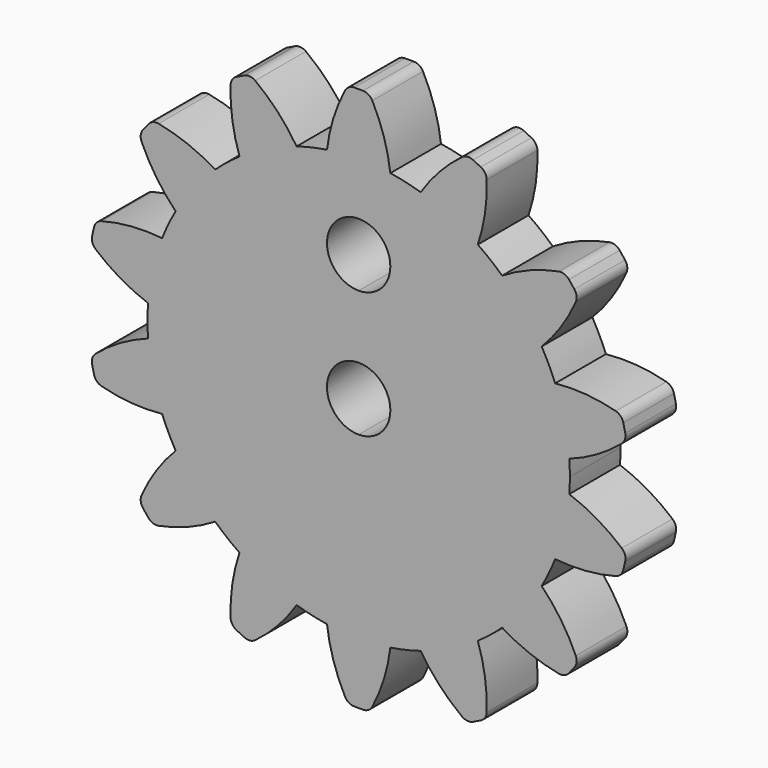
from build123d import *

# Parameters (mm, degrees)
F1_DEPTH = 3
F2_R     = 0.5


# Not quite as in the source:
# - a feature names something its author has since deleted; it is built from what else it names


with BuildPart() as f1:
    # F0 (on Front) → F1 (new body)
    with BuildSketch(Plane.XZ):
        with BuildLine():
            ThreePointArc((9.9727571462, -0.7376414454), (9.9931869657, -0.3690721728), (10, 0))
            ThreePointArc((10, 0), (9.9931869657, 0.3690721728), (9.9727571462, 0.7376414454))
            ThreePointArc((9.9727571462, 0.7376414454), (9.7492791218, 2.2252093396), (9.3051943444, 3.6624251819))
            ThreePointArc((9.3051943444, 3.6624251819), (9.009688679, 4.3388373912), (8.6650930875, 4.9916091379))
            ThreePointArc((8.6650930875, 4.9916091379), (7.8183148247, 6.2348980186), (6.7946236819, 7.3371035853))
            ThreePointArc((6.7946236819, 7.3371035853), (6.2348980186, 7.8183148247), (5.6412010723, 8.2569274226))
            ThreePointArc((5.6412010723, 8.2569274226), (4.3388373912, 9.009688679), (2.9382944686, 9.5585786399))
            ThreePointArc((2.9382944686, 9.5585786399), (2.2252093396, 9.7492791218), (1.5, 9.8868599666))
            ThreePointArc((1.5, 9.8868599666), (0, 10), (-1.5, 9.8868599666))
            ThreePointArc((-1.5, 9.8868599666), (-2.2252093396, 9.7492791218), (-2.9382944686, 9.5585786399))
            ThreePointArc((-2.9382944686, 9.5585786399), (-4.3388373912, 9.009688679), (-5.6412010723, 8.2569274226))
            ThreePointArc((-5.6412010723, 8.2569274226), (-6.2348980186, 7.8183148247), (-6.7946236819, 7.3371035853))
            ThreePointArc((-6.7946236819, 7.3371035853), (-7.8183148247, 6.2348980186), (-8.6650930875, 4.9916091379))
            ThreePointArc((-8.6650930875, 4.9916091379), (-9.009688679, 4.3388373912), (-9.3051943444, 3.6624251819))
            ThreePointArc((-9.3051943444, 3.6624251819), (-9.7492791218, 2.2252093396), (-9.9727571462, 0.7376414454))
            ThreePointArc((-9.9727571462, 0.7376414454), (-10, 0), (-9.9727571462, -0.7376414454))
            ThreePointArc((-9.9727571462, -0.7376414454), (-9.7492791218, -2.2252093396), (-9.3051943444, -3.6624251819))
            ThreePointArc((-9.3051943444, -3.6624251819), (-9.009688679, -4.3388373912), (-8.6650930875, -4.9916091379))
            ThreePointArc((-8.6650930875, -4.9916091379), (-7.8183148247, -6.2348980186), (-6.7946236819, -7.3371035853))
            ThreePointArc((-6.7946236819, -7.3371035853), (-6.2348980186, -7.8183148247), (-5.6412010723, -8.2569274226))
            ThreePointArc((-5.6412010723, -8.2569274226), (-4.3388373912, -9.009688679), (-2.9382944686, -9.5585786399))
            ThreePointArc((-2.9382944686, -9.5585786399), (-2.2252093396, -9.7492791218), (-1.5, -9.8868599666))
            ThreePointArc((-1.5, -9.8868599666), (0, -10), (1.5, -9.8868599666))
            ThreePointArc((1.5, -9.8868599666), (2.2252093396, -9.7492791218), (2.9382944686, -9.5585786399))
            ThreePointArc((2.9382944686, -9.5585786399), (4.3388373912, -9.009688679), (5.6412010723, -8.2569274226))
            ThreePointArc((5.6412010723, -8.2569274226), (6.2348980186, -7.8183148247), (6.7946236819, -7.3371035853))
            ThreePointArc((6.7946236819, -7.3371035853), (7.8183148247, -6.2348980186), (8.6650930875, -4.9916091379))
            ThreePointArc((8.6650930875, -4.9916091379), (9.009688679, -4.3388373912), (9.3051943444, -3.6624251819))
            ThreePointArc((9.3051943444, -3.6624251819), (9.7492791218, -2.2252093396), (9.9727571462, -0.7376414454))
        make_face()
        with BuildLine():
            ThreePointArc((0, 1.5), (1.0606601718, 1.0606601718), (1.5, 0))
            ThreePointArc((1.5, 0), (1.0606601718, -1.0606601718), (0, -1.5))
            ThreePointArc((0, -1.5), (-1.5, 0), (0, 1.5))
        make_face(mode=Mode.SUBTRACT)
        with BuildLine():
            ThreePointArc((1.5, 6), (1.0606601718, 4.9393398282), (0, 4.5))
            ThreePointArc((0, 4.5), (-1.0606601718, 7.0606601718), (1.5, 6))
        make_face(mode=Mode.SUBTRACT)
        with BuildLine():
            ThreePointArc((-5.6412010723, 8.2569274226), (-4.3388373912, 9.009688679), (-2.9382944686, 9.5585786399))
            ThreePointArc((-2.9382944686, 9.5585786399), (-3.9281759427, 10.8096541208), (-5.1466158007, 11.8394402655))
            Line((-5.1466158007, 11.8394402655), (-6.0475846686, 11.4055565264))
            ThreePointArc((-6.0475846686, 11.4055565264), (-6.002150266, 9.8108807266), (-5.6412010723, 8.2569274226))
        make_face()
        with BuildLine():
            ThreePointArc((-1.5, 9.8868599666), (0, 10), (1.5, 9.8868599666))
            ThreePointArc((1.5, 9.8868599666), (1.1509689165, 11.4435335015), (0.5, 12.9))
            Line((0.5, 12.9), (-0.5, 12.9))
            ThreePointArc((-0.5, 12.9), (-1.1509689165, 11.4435335015), (-1.5, 9.8868599666))
        make_face()
        with BuildLine():
            ThreePointArc((-8.6650930875, 4.9916091379), (-7.8183148247, 6.2348980186), (-6.7946236819, 7.3371035853))
            ThreePointArc((-6.7946236819, 7.3371035853), (-8.2292973805, 8.0347901697), (-9.7738812229, 8.4339341852))
            Line((-9.7738812229, 8.4339341852), (-10.3973710248, 7.6521027027))
            ThreePointArc((-10.3973710248, 7.6521027027), (-9.6645321438, 6.2350627012), (-8.6650930875, 4.9916091379))
        make_face()
        with BuildLine():
            ThreePointArc((-9.9727571462, 0.7376414454), (-9.7492791218, 2.2252093396), (-9.3051943444, 3.6624251819))
            ThreePointArc((-9.3051943444, 3.6624251819), (-10.9005055464, 3.6685374852), (-12.4653096002, 3.3579840041))
            Line((-12.4653096002, 3.3579840041), (-12.6878305341, 2.3830560919))
            ThreePointArc((-12.6878305341, 2.3830560919), (-11.4127349029, 1.4243140398), (-9.9727571462, 0.7376414454))
        make_face()
        with BuildLine():
            ThreePointArc((-12.4653096002, -3.3579840041), (-10.9005055464, -3.6685374852), (-9.3051943444, -3.6624251819))
            ThreePointArc((-9.3051943444, -3.6624251819), (-9.7492791218, -2.2252093396), (-9.9727571462, -0.7376414454))
            ThreePointArc((-9.9727571462, -0.7376414454), (-11.4127349029, -1.4243140398), (-12.6878305341, -2.3830560919))
            Line((-12.6878305341, -2.3830560919), (-12.4653096002, -3.3579840041))
        make_face()
        with BuildLine():
            ThreePointArc((-9.7738812229, -8.4339341852), (-8.2292973805, -8.0347901697), (-6.7946236819, -7.3371035853))
            ThreePointArc((-6.7946236819, -7.3371035853), (-7.8183148247, -6.2348980186), (-8.6650930875, -4.9916091379))
            ThreePointArc((-8.6650930875, -4.9916091379), (-9.6645321438, -6.2350627012), (-10.3973710248, -7.6521027027))
            Line((-10.3973710248, -7.6521027027), (-9.7738812229, -8.4339341852))
        make_face()
        with BuildLine():
            ThreePointArc((-5.1466158007, -11.8394402655), (-3.9281759427, -10.8096541208), (-2.9382944686, -9.5585786399))
            ThreePointArc((-2.9382944686, -9.5585786399), (-4.3388373912, -9.009688679), (-5.6412010723, -8.2569274226))
            ThreePointArc((-5.6412010723, -8.2569274226), (-6.002150266, -9.8108807266), (-6.0475846686, -11.4055565264))
            Line((-6.0475846686, -11.4055565264), (-5.1466158007, -11.8394402655))
        make_face()
        with BuildLine():
            ThreePointArc((0.5, -12.9), (1.1509689165, -11.4435335015), (1.5, -9.8868599666))
            ThreePointArc((1.5, -9.8868599666), (0, -10), (-1.5, -9.8868599666))
            ThreePointArc((-1.5, -9.8868599666), (-1.1509689165, -11.4435335015), (-0.5, -12.9))
            Line((-0.5, -12.9), (0.5, -12.9))
        make_face()
        with BuildLine():
            ThreePointArc((6.0475846686, -11.4055565264), (6.002150266, -9.8108807266), (5.6412010723, -8.2569274226))
            ThreePointArc((5.6412010723, -8.2569274226), (4.3388373912, -9.009688679), (2.9382944686, -9.5585786399))
            ThreePointArc((2.9382944686, -9.5585786399), (3.9281759427, -10.8096541208), (5.1466158007, -11.8394402655))
            Line((5.1466158007, -11.8394402655), (6.0475846686, -11.4055565264))
        make_face()
        with BuildLine():
            ThreePointArc((10.3973710248, -7.6521027027), (9.6645321438, -6.2350627012), (8.6650930875, -4.9916091379))
            ThreePointArc((8.6650930875, -4.9916091379), (7.8183148247, -6.2348980186), (6.7946236819, -7.3371035853))
            ThreePointArc((6.7946236819, -7.3371035853), (8.2292973805, -8.0347901697), (9.7738812229, -8.4339341852))
            Line((9.7738812229, -8.4339341852), (10.3973710248, -7.6521027027))
        make_face()
        with BuildLine():
            ThreePointArc((12.6878305341, -2.3830560919), (11.4127349029, -1.4243140398), (9.9727571462, -0.7376414454))
            ThreePointArc((9.9727571462, -0.7376414454), (9.7492791218, -2.2252093396), (9.3051943444, -3.6624251819))
            ThreePointArc((9.3051943444, -3.6624251819), (10.9005055464, -3.6685374852), (12.4653096002, -3.3579840041))
            Line((12.4653096002, -3.3579840041), (12.6878305341, -2.3830560919))
        make_face()
        with BuildLine():
            ThreePointArc((9.3051943444, 3.6624251819), (9.7492791218, 2.2252093396), (9.9727571462, 0.7376414454))
            ThreePointArc((9.9727571462, 0.7376414454), (11.4127349029, 1.4243140398), (12.6878305341, 2.3830560919))
            Line((12.6878305341, 2.3830560919), (12.4653096002, 3.3579840041))
            ThreePointArc((12.4653096002, 3.3579840041), (10.9005055464, 3.6685374852), (9.3051943444, 3.6624251819))
        make_face()
        with BuildLine():
            ThreePointArc((6.7946236819, 7.3371035853), (7.8183148247, 6.2348980186), (8.6650930875, 4.9916091379))
            ThreePointArc((8.6650930875, 4.9916091379), (9.6645321438, 6.2350627012), (10.3973710248, 7.6521027027))
            Line((10.3973710248, 7.6521027027), (9.7738812229, 8.4339341852))
            ThreePointArc((9.7738812229, 8.4339341852), (8.2292973805, 8.0347901697), (6.7946236819, 7.3371035853))
        make_face()
        with BuildLine():
            ThreePointArc((2.9382944686, 9.5585786399), (4.3388373912, 9.009688679), (5.6412010723, 8.2569274226))
            ThreePointArc((5.6412010723, 8.2569274226), (6.002150266, 9.8108807266), (6.0475846686, 11.4055565264))
            Line((6.0475846686, 11.4055565264), (5.1466158007, 11.8394402655))
            ThreePointArc((5.1466158007, 11.8394402655), (3.9281759427, 10.8096541208), (2.9382944686, 9.5585786399))
        make_face()
    extrude(amount=F1_DEPTH)

    # F2
    f2_edges = [f1.edges().sort_by_distance(p)[0] for p in [
        (-5.146616, -1.5, 11.83944),
        (-6.047585, -1.5, 11.405557),
        (-9.773881, -1.5, 8.433934),
        (-10.397371, -1.5, 7.652103),
        (-0.5, -1.5, 12.9),
        (0.5, -1.5, 12.9),
        (5.146616, -1.5, 11.83944),
        (6.047585, -1.5, 11.405557),
        (9.773881, -1.5, 8.433934),
        (10.397371, -1.5, 7.652103),
        (12.46531, -1.5, 3.357984),
        (12.687831, -1.5, 2.383056),
        (12.687831, -1.5, -2.383056),
        (12.46531, -1.5, -3.357984),
        (10.397371, -1.5, -7.652103),
        (9.773881, -1.5, -8.433934),
        (6.047585, -1.5, -11.405557),
        (5.146616, -1.5, -11.83944),
        (0.5, -1.5, -12.9),
        (-0.5, -1.5, -12.9),
        (-5.146616, -1.5, -11.83944),
        (-6.047585, -1.5, -11.405557),
        (-12.46531, -1.5, 3.357984),
        (-12.687831, -1.5, 2.383056),
        (-12.687831, -1.5, -2.383056),
        (-12.46531, -1.5, -3.357984),
        (-9.773881, -1.5, -8.433934),
        (-10.397371, -1.5, -7.652103),
    ]]
    fillet(f2_edges, radius=F2_R)


solid = f1.part
